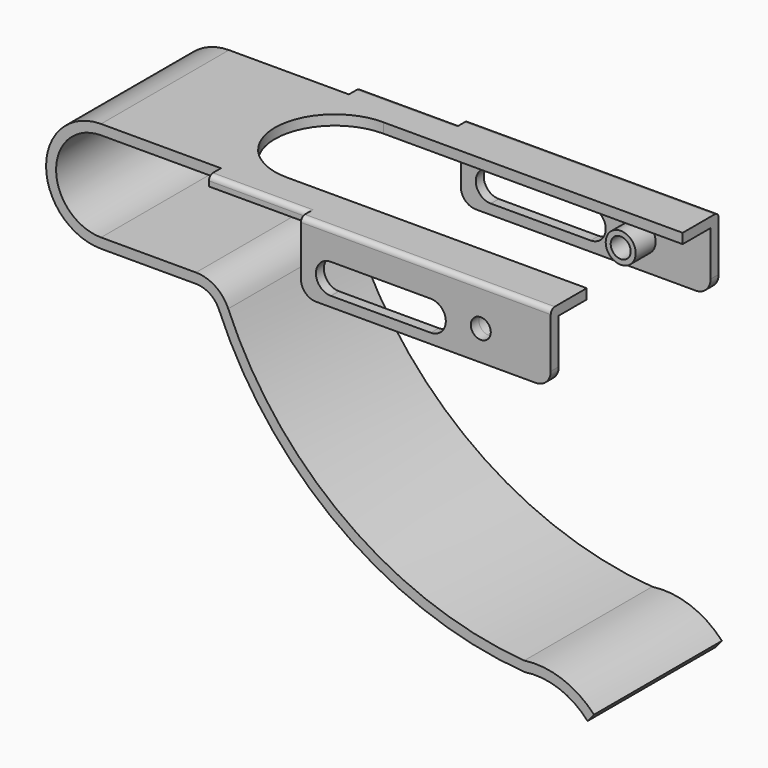
from build123d import *

# Parameters (mm, degrees)
F1_DEPTH  = 16
F2_W      = 70
F2_H      = 3
F3_DEPTH  = 2
F4_W      = 50
F4_H      = 14
F5_DEPTH  = 2
F6_R      = 1
F9_DEPTH  = 2
F11_DEPTH = 42.001
F13_D     = 4
F14_R     = 3
F14_R_2   = 2
F15_DEPTH = 5
F16_R     = 3


# Not quite as in the source:
# - a pattern or mirror of a feature is missing from the dataset's text; its kind, count and spacing are read off the source's solid


with BuildPart() as f1:
    # F0 (on Front) → F1 (new body)
    with BuildSketch(Plane.XZ):
        with BuildLine():
            Line((94, 11), (0, 11))
            ThreePointArc((0, 11), (-11, 0), (0, -11))
            Line((0, -11), (19, -11))
            ThreePointArc((19, -11), (21.7681124643, -11.8361612201), (23.6103896104, -14.064978646))
            ThreePointArc((23.6103896104, -14.064978646), (47.9882051962, -44.6729645648), (84.7744660979, -58.0107943585))
            ThreePointArc((84.7744660979, -58.0107943585), (91.6454906811, -58.677418602), (97.362645896, -62.5464627931))
            Line((97.362645896, -62.5464627931), (98.6602822553, -61))
            ThreePointArc((98.6602822553, -61), (92.2959119196, -56.7859373435), (84.7034264019, -56))
            ThreePointArc((84.7034264019, -56), (49.0672193413, -42.9854179344), (25.4545454545, -13.2909701044))
            ThreePointArc((25.4545454545, -13.2909701044), (22.87535745, -10.1706257081), (19, -9))
            Line((19, -9), (0, -9))
            ThreePointArc((0, -9), (-9, 0), (0, 9))
            Line((0, 9), (94, 9))
            Line((94, 9), (94, 11))
        make_face()
    extrude(amount=F1_DEPTH)

    # F2 (on face) → F3 (join)
    with BuildSketch(Plane.XY.offset(11)):
        with Locations((59, -17.5)):
            Rectangle(F2_W, F2_H)
    extrude(amount=-F3_DEPTH)

    # F4 (on face) → F5 (join)
    with BuildSketch(Plane.XZ.offset(19)):
        with Locations((69, 4)):
            Rectangle(F4_W, F4_H)
    extrude(amount=F5_DEPTH)

    # F6
    f6_edges = [f1.edges().sort_by_distance(p)[0] for p in [
        (69, -21, 11),
        (34, -19, 11),
    ]]
    fillet(f6_edges, radius=F6_R)

    # F7: F1 across plane


with BuildPart() as f1_1:
    add(f1.part)
    add(f1.part.mirror(Plane.XZ))

    # F8 (on face) → F9 (cut)
    with BuildSketch(Plane.XY.offset(11)):
        with BuildLine():
            Line((94, 11.9996714485), (34.088798243, 11.9996714485))
            ThreePointArc((34.088798243, 11.9996714485), (22.0000004897, -0.003428249), (34.0956545385, -11.9996187527))
            Line((34.0956545385, -11.9996187527), (94, -11.9996187527))
            Line((94, -11.9996187527), (94, 11.9996714485))
        make_face()
    extrude(amount=-F9_DEPTH, mode=Mode.SUBTRACT)

    # F10 (on face) → F11 (cut, through all)
    with BuildSketch(Plane.XZ.offset(21)):
        with BuildLine():
            ThreePointArc((50, 5), (47, 2), (50, -1))
            Line((50, -1), (70, -1))
            ThreePointArc((70, -1), (73, 2), (70, 5))
            Line((70, 5), (50, 5))
        make_face()
    extrude(amount=-F11_DEPTH, mode=Mode.SUBTRACT)

    # F13 (through all)
    with Locations(Plane.XZ.offset(21)):
        with Locations((80, 3)):
            Hole(F13_D / 2)

    # F14 (on face) → F15 (join)
    with BuildSketch(Plane(origin=(0, -19, 0), x_dir=(-1, 0, 0), z_dir=(0, 1, 0))):
        with Locations((-80, 3)):
            Circle(F14_R)
        with Locations((-80, 3)):
            Circle(F14_R_2, mode=Mode.SUBTRACT)
    f15 = extrude(amount=F15_DEPTH)

    # F15_copies: F15 across plane
    add(f15.mirror(Plane.ZX))

    # F16
    f16_edges = [f1_1.edges().sort_by_distance(p)[0] for p in [
        (44, 20, -3),
        (94, 20, -3),
        (94, -20, -3),
        (44, -20, -3),
    ]]
    fillet(f16_edges, radius=F16_R)


solid = f1_1.part
